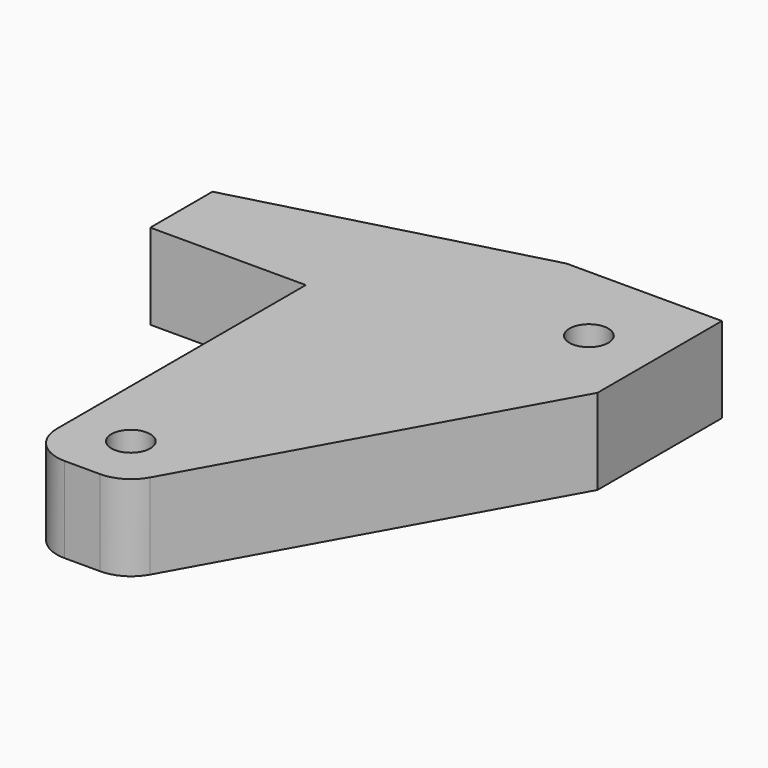
from build123d import *

# Parameters (mm, degrees)
F0_W      = 15
F0_H      = 18
F1_DEPTH  = 4.4
F2_R      = 2
F3_SIZE2  = 9.99999
F3_SIZE   = 17.99999
F4_R      = 2
F6_W      = 8
F6_H      = 4.4
F6_W_2    = 15
F7_DEPTH  = 4
F8_DEPTH  = 4
F9_SIZE2  = 15
F9_SIZE   = 4
F10_DEPTH = 4.4
F11_R     = 1
F12_DEPTH = 4.4


# Not quite as in the source:
# - a fillet or chamfer is up to 0.001 mm smaller than in the source, because OpenCascade refuses the exact size


with BuildPart() as f1:
    # F0 (on Top) → F1 (new body)
    with BuildSketch(Plane.XY):
        with Locations((7.5, 9)):
            Rectangle(F0_W, F0_H)
    extrude(amount=F1_DEPTH)

    # F2
    f2_edges = [f1.edges().sort_by_distance(p)[0] for p in [
        (0, 0, 2.2),
    ]]
    fillet(f2_edges, radius=F2_R)

    # F3 (size 18 and 10 in the source; OpenCascade refuses exactly that, so slightly less here)
    f3_edges = [f1.edges().sort_by_distance(p)[0] for p in [
        (15, 0, 2.2),
    ]]
    f3_side = f1.faces().sort_by_distance((15, 9, 2.2))[0]
    chamfer(f3_edges, length=F3_SIZE, length2=F3_SIZE2, reference=f3_side)

    # F4
    f4_edges = [f1.edges().sort_by_distance(p)[0] for p in [
        (5.00001, 0, 2.2),
    ]]
    fillet(f4_edges, radius=F4_R)

    # F6 (on face) → F7 (join)
    with BuildSketch(Plane(origin=(0, 18, 0), x_dir=(-1, 0, 0), z_dir=(0, 1, 0))):
        with Locations((4, 2.2)):
            Rectangle(F6_W, F6_H)
        with Locations((-7.5, 2.2)):
            Rectangle(F6_W_2, F6_H)
    extrude(amount=F7_DEPTH)

    # F8 (add): a face of the model
    f8_faces = [f1.faces().sort_by_distance(p)[0] for p in [
        (3.5, 22, 2.2),
    ]]
    extrude(f8_faces, amount=F8_DEPTH)

    # F9
    f9_edges = [f1.edges().sort_by_distance(p)[0] for p in [
        (-8, 26, 2.2),
    ]]
    f9_side = f1.faces().sort_by_distance((-8, 22, 2.2))[0]
    chamfer(f9_edges, length=F9_SIZE, length2=F9_SIZE2, reference=f9_side)

    # F5 (on face) → F10 (cut)
    with BuildSketch(Plane(origin=(0, 0, 0), x_dir=(1, 0, 0), z_dir=(0, 0, -1))):
        with BuildLine():
            ThreePointArc((2, -3), (3, -4), (4, -3))
            ThreePointArc((4, -3), (3, -2), (2, -3))
        make_face()
    extrude(amount=-F10_DEPTH, mode=Mode.SUBTRACT)

    # F11 (on face) → F12 (cut)
    with BuildSketch(Plane(origin=(0, 0, 0), x_dir=(1, 0, 0), z_dir=(0, 0, -1))):
        with Locations((11.6287460551, -21.6625984758)):
            Circle(F11_R)
    extrude(amount=-F12_DEPTH, mode=Mode.SUBTRACT)


solid = f1.part
